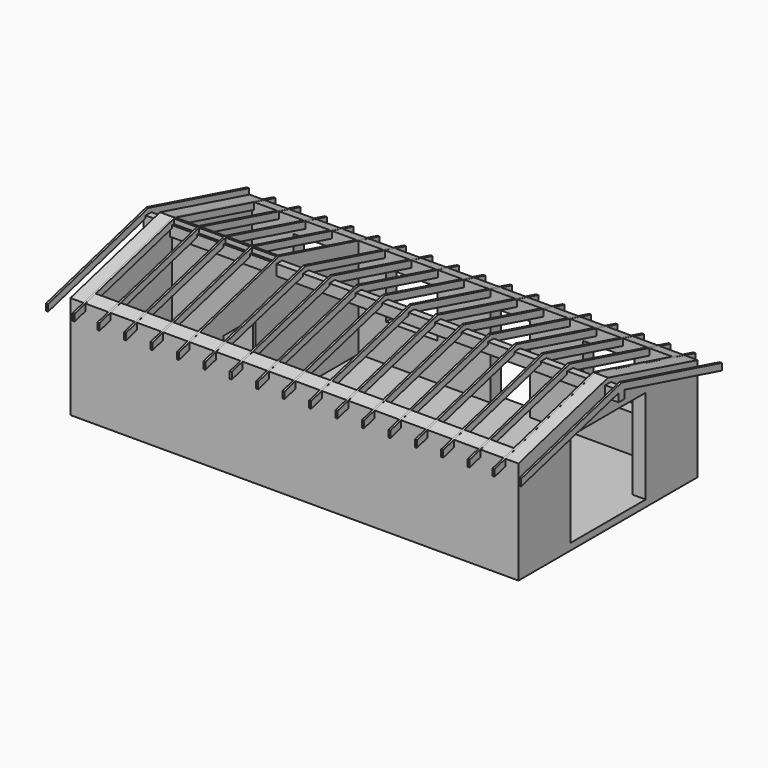
from build123d import *

# Parameters (mm, degrees)
F0_W           = 254
F0_H           = 127
F0_W_2         = 59.1058
F0_H_2         = 55.499
F0_H_3         = 55.626
F0_W_3         = 179.0192
F0_H_4         = 112.268
F1_DEPTH       = 3.81
F2_DEPTH       = 76.2
F4_DEPTH       = 254
F3_W           = 53.34
F3_H           = 53.34
F5_DEPTH       = 7.366
F7_START       = -119.38
F6_W           = 29.083
F6_H           = 26.797
F6_W_2         = 22.606
F6_H_2         = 48.006
F7_DEPTH       = 7.62
F8_W           = 22.606
F8_H           = 48.006
F9_DEPTH       = 1.27
F3_W_2         = 4.064
F3_H_2         = 6.096
F10_DEPTH      = 261.62
F10_DEPTH_BACK = 7.62
F11_W          = 1.143
F11_H          = 83.82
F12_DEPTH      = 3.683
F12_DEPTH_BACK = 0.0254
F14_DEPTH      = 271.78
F15_W          = 1.143
F15_H          = 83.82
F16_DEPTH      = 3.683
F16_DEPTH_BACK = 0.0254
F18_DEPTH      = 271.78


# Not quite as in the source:
# - a feature names something its author has since deleted; it is built from what else it names


with BuildPart() as f1:
    # F0 (on Top) → F1 (new body)
    with BuildSketch(Plane.XY):
        with Locations((-127, 63.5)):
            Rectangle(F0_W, F0_H)
        with Locations((-217.0811, 35.1155)):
            Rectangle(F0_W_2, F0_H_2, mode=Mode.SUBTRACT)
        with Locations((-217.0811, 91.821)):
            Rectangle(F0_W_2, F0_H_3, mode=Mode.SUBTRACT)
        with Locations((-96.8756, 63.5)):
            Rectangle(F0_W_3, F0_H_4, mode=Mode.SUBTRACT)
        with Locations((-96.8756, 63.5)):
            Rectangle(F0_W_3, F0_H_4)
        with Locations((-217.0811, 91.821)):
            Rectangle(F0_W_2, F0_H_3)
        with Locations((-217.0811, 35.1155)):
            Rectangle(F0_W_2, F0_H_2)
    extrude(amount=F1_DEPTH)

    # F0 (on Top) → F2 (join)
    with BuildSketch(Plane.XY):
        with Locations((-127, 63.5)):
            Rectangle(F0_W, F0_H)
        with Locations((-217.0811, 35.1155)):
            Rectangle(F0_W_2, F0_H_2, mode=Mode.SUBTRACT)
        with Locations((-217.0811, 91.821)):
            Rectangle(F0_W_2, F0_H_3, mode=Mode.SUBTRACT)
        with Locations((-96.8756, 63.5)):
            Rectangle(F0_W_3, F0_H_4, mode=Mode.SUBTRACT)
    extrude(amount=F2_DEPTH)

    # F3 (on Right) → F4 (cut)
    with BuildSketch(Plane.YZ):
        Polygon((0, 83.7605968118), (0, 58.42), (63.5, 75.4347737194), (127, 58.42), (127, 83.7605968118), align=None)
    extrude(amount=-F4_DEPTH, mode=Mode.SUBTRACT)

    # F3 (on Right) → F5 (cut)
    with BuildSketch(Plane.YZ):
        with Locations((63.5, 30.48)):
            Rectangle(F3_W, F3_H)
    extrude(amount=-F5_DEPTH, mode=Mode.SUBTRACT)

    # F6 (on Front) → F7 (cut)
    with BuildSketch(Plane.XZ.offset(F7_START)):
        with Locations((-44.5135, 38.4175)):
            Rectangle(F6_W, F6_H)
        with Locations((-100.33, 27.813)):
            Rectangle(F6_W_2, F6_H_2)
        with Locations((-156.1465, 38.4175)):
            Rectangle(F6_W, F6_H)
        with Locations((-211.963, 27.813)):
            Rectangle(F6_W_2, F6_H_2)
    extrude(amount=-F7_DEPTH, mode=Mode.SUBTRACT)

    # F8 (on face) → F9 (cut)
    with BuildSketch(Plane.YZ.offset(-186.3852)):
        with Locations((35.179, 27.813)):
            Rectangle(F8_W, F8_H)
    extrude(amount=-F9_DEPTH, mode=Mode.SUBTRACT)

    # F3 (on Right) → F10 (join, two sides)
    with BuildSketch(Plane.YZ) as f10_sk:
        with Locations((63.5, 69.4756596119)):
            Rectangle(F3_W_2, F3_H_2)
    extrude(amount=-F10_DEPTH)
    extrude(f10_sk.sketch, amount=F10_DEPTH_BACK)

    # F11 (on face) → F12 (join, two sides)
    with BuildSketch(Plane(origin=(0, 23.1123868597, 86.2566020445), x_dir=(1, 0, 0), z_dir=(0, 0.2588190451, 0.9659258263))) as f12_sk:
        with Locations((7.0485, 83.7223338678)):
            Rectangle(F11_W, F11_H)
        with Locations((-7.9375, 83.7223338678)):
            Rectangle(F11_W, F11_H)
        with Locations((-22.1107, 83.7223338678)):
            Rectangle(F11_W, F11_H)
        with Locations((-37.0967, 83.7223338678)):
            Rectangle(F11_W, F11_H)
        with Locations((-52.0827, 83.7223338678)):
            Rectangle(F11_W, F11_H)
        with Locations((-67.0687, 83.7223338678)):
            Rectangle(F11_W, F11_H)
        with Locations((-82.0547, 83.7223338678)):
            Rectangle(F11_W, F11_H)
        with Locations((-97.0407, 83.7223338678)):
            Rectangle(F11_W, F11_H)
        with Locations((-112.0267, 83.7223338678)):
            Rectangle(F11_W, F11_H)
        with Locations((-127.0127, 83.7223338678)):
            Rectangle(F11_W, F11_H)
        with Locations((-141.9987, 83.7223338678)):
            Rectangle(F11_W, F11_H)
        with Locations((-156.9847, 83.7223338678)):
            Rectangle(F11_W, F11_H)
        with Locations((-171.9707, 83.7223338678)):
            Rectangle(F11_W, F11_H)
        with Locations((-186.9567, 83.7223338678)):
            Rectangle(F11_W, F11_H)
        with Locations((-201.9427, 83.7223338678)):
            Rectangle(F11_W, F11_H)
        with Locations((-216.9287, 83.7223338678)):
            Rectangle(F11_W, F11_H)
        with Locations((-231.9147, 83.7223338678)):
            Rectangle(F11_W, F11_H)
        with Locations((-246.0625, 83.7223338678)):
            Rectangle(F11_W, F11_H)
        with Locations((-261.0993, 83.7223338678)):
            Rectangle(F11_W, F11_H)
    extrude(amount=-F12_DEPTH)
    extrude(f12_sk.sketch, amount=F12_DEPTH_BACK)

    # F13 (on face) → F14 (cut)
    with BuildSketch(Plane.YZ.offset(7.62)):
        Polygon((146.9239283621, 53.1076955003), (134.6566703682, 56.3946973731), (134.6566703682, 52.5554791857), (146.9239283621, 49.2684773129), align=None)
    extrude(amount=-F14_DEPTH, mode=Mode.SUBTRACT)

    # F15 (on face) → F16 (join, two sides)
    with BuildSketch(Plane(origin=(0, -14.605, 54.5066020445), x_dir=(1, 0, 0), z_dir=(0, -0.2588190451, 0.9659258263))) as f16_sk:
        with Locations((7.0485, 38.9502460709)):
            Rectangle(F15_W, F15_H)
        with Locations((-7.9375, 38.9502460709)):
            Rectangle(F15_W, F15_H)
        with Locations((-22.1107, 38.9502460709)):
            Rectangle(F15_W, F15_H)
        with Locations((-37.0967, 38.9502460709)):
            Rectangle(F15_W, F15_H)
        with Locations((-52.0827, 38.9502460709)):
            Rectangle(F15_W, F15_H)
        with Locations((-67.0687, 38.9502460709)):
            Rectangle(F15_W, F15_H)
        with Locations((-82.0547, 38.9502460709)):
            Rectangle(F15_W, F15_H)
        with Locations((-97.0407, 38.9502460709)):
            Rectangle(F15_W, F15_H)
        with Locations((-112.0267, 38.9502460709)):
            Rectangle(F15_W, F15_H)
        with Locations((-127.0127, 38.9502460709)):
            Rectangle(F15_W, F15_H)
        with Locations((-141.9987, 38.9502460709)):
            Rectangle(F15_W, F15_H)
        with Locations((-156.9847, 38.9502460709)):
            Rectangle(F15_W, F15_H)
        with Locations((-171.9707, 38.9502460709)):
            Rectangle(F15_W, F15_H)
        with Locations((-186.9567, 38.9502460709)):
            Rectangle(F15_W, F15_H)
        with Locations((-201.9427, 38.9502460709)):
            Rectangle(F15_W, F15_H)
        with Locations((-216.9287, 38.9502460709)):
            Rectangle(F15_W, F15_H)
        with Locations((-231.9147, 38.9502460709)):
            Rectangle(F15_W, F15_H)
        with Locations((-246.0625, 38.9502460709)):
            Rectangle(F15_W, F15_H)
        with Locations((-261.0993, 38.9502460709)):
            Rectangle(F15_W, F15_H)
    extrude(amount=-F16_DEPTH)
    extrude(f16_sk.sketch, amount=F16_DEPTH_BACK)

    # F17 (on face) → F18 (cut)
    with BuildSketch(Plane.YZ.offset(7.62)):
        Polygon((-7.6444030343, 52.5587662079), (-7.6444030343, 56.3979843953), (-19.9116610281, 53.1109825225), (-19.9116610281, 49.2717643351), align=None)
    extrude(amount=-F18_DEPTH, mode=Mode.SUBTRACT)


solid = f1.part
